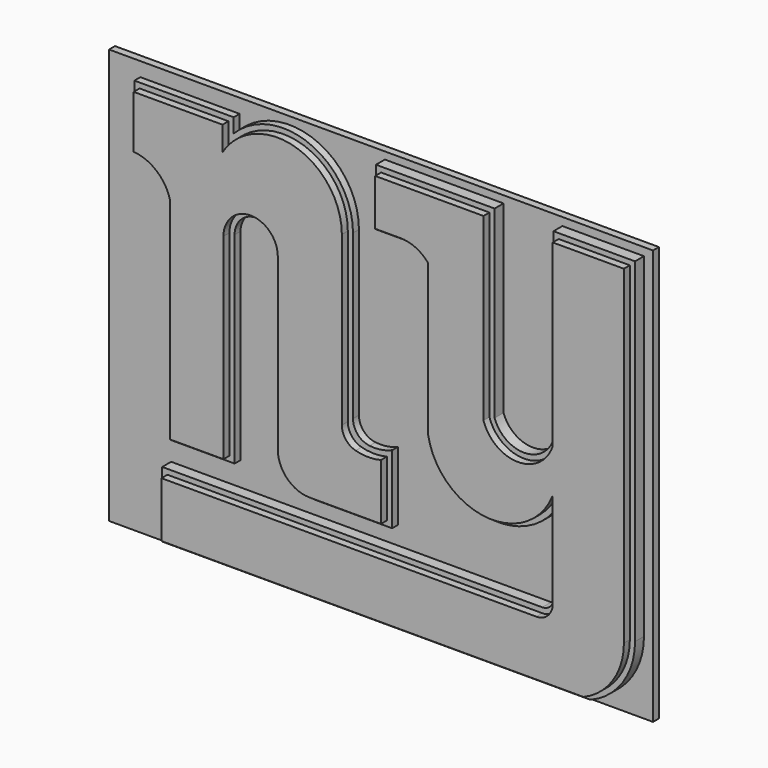
from build123d import *

# Parameters (mm, degrees)
F1_DEPTH = 3.81
F2_W     = 185.822121799
F2_H     = 141.7885944247
F3_DEPTH = 2.54
F5_DEPTH = 2.54
F7_DEPTH = 2.54
F9_DEPTH = 2.54


# Not quite as in the source:
# - a feature names something its author has since deleted; it is built from what else it names


with BuildPart() as f1:
    # F0 (on Front) → F1 (new body)
    with BuildSketch(Plane.XZ):
        with BuildLine():
            Line((61.8872972369, -59.9267967045), (-67.9568648338, -59.9267967045))
            Line((-67.9568648338, -59.9267967045), (-67.9568648338, -82.3878794909))
            Line((-67.9568648338, -82.3878794909), (78.2999321818, -82.3878794909))
            ThreePointArc((78.2999321818, -82.3878794909), (89.3836158058, -73.5038786726), (93.5593023896, -59.9267967045))
            Line((93.5593023896, -59.9267967045), (93.5593023896, 54.4298999012))
            Line((93.5593023896, 54.4298999012), (65.6972972369, 54.4298999012))
            Line((65.6972972369, 54.4298999012), (65.6972972369, -8.2891006023))
            ThreePointArc((65.6972972369, -8.2891006023), (55.6403416055, -15.4575892654), (45.5833859742, -8.2891006023))
            Line((45.5833859742, -8.2891006023), (45.5833859742, 54.7044351697))
            Line((45.5833859742, 54.7044351697), (5.0396709703, 54.7044351697))
            Line((5.0396709703, 54.7044351697), (5.0396709703, 35.2702587843))
            Line((5.0396709703, 35.2702587843), (15.4831645885, 35.2702587843))
            ThreePointArc((15.4831645885, 35.2702587843), (19.6591632782, 34.3958519091), (23.1335591525, 31.9195389748))
            Line((23.1335591525, 31.9195389748), (23.1335591525, -17.3360444605))
            Line((23.1335591525, -17.3360444605), (23.1335591525, -19.20456164))
            ThreePointArc((23.1335591525, -19.20456164), (40.879363735, -38.4902332098), (65.6972972369, -30.0687793642))
            Line((65.6972972369, -30.0687793642), (65.6972972369, -56.1167967045))
            ThreePointArc((65.6972972369, -56.1167967045), (64.5813740732, -58.8108735409), (61.8872972369, -59.9267967045))
        make_face()
        with BuildLine():
            ThreePointArc((23.1335591525, -17.3360444605), (23.1145151518, -18.2703030503), (23.1335591525, -19.20456164))
            Line((23.1335591525, -19.20456164), (23.1335591525, -17.3360444605))
        make_face()
    extrude(amount=F1_DEPTH)

    # F8 (on face) → F9 (join)
    with BuildSketch(Plane.XZ.offset(3.81)):
        with BuildLine():
            Line((67.4725060976, -23.4798739041), (67.4725060976, -56.1167967045))
            ThreePointArc((67.4725060976, -56.1167967045), (65.8366362966, -60.0661357642), (61.8872972369, -61.7020055652))
            Line((61.8872972369, -61.7020055652), (-66.1816559732, -61.7020055652))
            Line((-66.1816559732, -61.7020055652), (-66.1816559732, -80.6126706302))
            Line((-66.1816559732, -80.6126706302), (77.9542927434, -80.6126706302))
            ThreePointArc((77.9542927434, -80.6126706302), (88.0081874746, -72.3683477517), (91.784093529, -59.9267967045))
            Line((91.784093529, -59.9267967045), (91.784093529, 52.6546910405))
            Line((91.784093529, 52.6546910405), (67.4725060976, 52.6546910405))
            Line((67.4725060976, 52.6546910405), (67.4725060976, -8.5750017462))
            ThreePointArc((67.4725060976, -8.5750017462), (55.6403416055, -17.2327981261), (43.8081771135, -8.5750017462))
            Line((43.8081771135, -8.5750017462), (43.8081771135, 52.9292263091))
            Line((43.8081771135, 52.9292263091), (6.8148798309, 52.9292263091))
            Line((6.8148798309, 52.9292263091), (6.8148798309, 37.0454676449))
            Line((6.8148798309, 37.0454676449), (15.4831645885, 37.0454676449))
            ThreePointArc((15.4831645885, 37.0454676449), (20.6976230432, 35.8732781186), (24.9087680131, 32.5822504214))
            Line((24.9087680131, 32.5822504214), (24.9087680131, -17.3729597743))
            ThreePointArc((24.9087680131, -17.3729597743), (24.8898523858, -18.1966120898), (24.9030282278, -19.0203762156))
            ThreePointArc((24.9030282278, -19.0203762156), (44.5022080749, -37.3401368279), (67.4725060976, -23.4798739041))
        make_face()
    extrude(amount=F9_DEPTH)


with BuildPart() as f3:
    # F2 (on face) → F3 (new body)
    with BuildSketch(Plane(origin=(0, 0, 0), x_dir=(-1, 0, 0), z_dir=(0, 1, 0))):
        with Locations((-3.7357322872, -13.7389265001)):
            Rectangle(F2_W, F2_H)
    extrude(amount=F3_DEPTH)

    # F4 (on face) → F5 (join)
    with BuildSketch(Plane.XZ):
        with BuildLine():
            Line((-66.1017629318, 21.9844542444), (-66.1017629318, -51.7266206443))
            Line((-66.1017629318, -51.7266206443), (-44.2493627779, -51.7266206443))
            Line((-44.2493627779, -51.7266206443), (-44.2493627779, 17.092127353))
            ThreePointArc((-44.2493627779, 17.092127353), (-36.7477941327, 24.5936959982), (-29.2462254874, 17.092127353))
            Line((-29.2462254874, 17.092127353), (-29.2462254874, -40.983552891))
            ThreePointArc((-29.2462254874, -40.983552891), (-25.5264816085, -49.9638090121), (-16.5462254874, -53.683552891))
            Line((-16.5462254874, -53.683552891), (9.566242341, -53.683552891))
            Line((9.566242341, -53.683552891), (9.566242341, -30.2003771067))
            ThreePointArc((9.566242341, -30.2003771067), (5.7901732638, -31.2942255388), (1.8598167011, -31.380824371))
            ThreePointArc((1.8598167011, -31.380824371), (-2.1819158801, -29.3091628597), (-3.8061193191, -25.0677778425))
            Line((-3.8061193191, -25.0677778425), (-3.8061193191, 30.7906456292))
            ThreePointArc((-3.8061193191, 30.7906456292), (-18.6015771181, 52.8067259199), (-44.5755193941, 47.4245622754))
            Line((-44.5755193941, 47.4245622754), (-44.5755193941, 52.3168891668))
            Line((-44.5755193941, 52.3168891668), (-78.4956621937, 52.3168891668))
            Line((-78.4956621937, 52.3168891668), (-78.4956621937, 30.7906456292))
            ThreePointArc((-78.4956621937, 30.7906456292), (-70.7684925993, 28.5411928963), (-66.1017629318, 21.9844542444))
        make_face()
    extrude(amount=F5_DEPTH)

    # F6 (on face) → F7 (join)
    with BuildSketch(Plane.XZ.offset(2.54)):
        with BuildLine():
            Line((-76.7176621937, 50.5388891668), (-76.7176621937, 32.5374547699))
            ThreePointArc((-76.7176621937, 32.5374547699), (-68.8934526322, 29.3403456584), (-64.3237629318, 22.2299520002))
            Line((-64.3237629318, 22.2299520002), (-64.3237629318, -49.9486206443))
            Line((-64.3237629318, -49.9486206443), (-46.0273627779, -49.9486206443))
            Line((-46.0273627779, -49.9486206443), (-46.0273627779, 17.092127353))
            ThreePointArc((-46.0273627779, 17.092127353), (-36.7477941327, 26.3716959982), (-27.4682254874, 17.092127353))
            Line((-27.4682254874, 17.092127353), (-27.4682254874, -40.983552891))
            ThreePointArc((-27.4682254874, -40.983552891), (-24.2692457516, -48.7065731551), (-16.5462254874, -51.905552891))
            Line((-16.5462254874, -51.905552891), (7.788242341, -51.905552891))
            Line((7.788242341, -51.905552891), (7.788242341, -32.6938578527))
            ThreePointArc((7.788242341, -32.6938578527), (3.4584477385, -33.2470515492), (-0.8690068072, -32.6758408003))
            ThreePointArc((-0.8690068072, -32.6758408003), (-4.2691980449, -30.4090810578), (-5.5841193191, -26.5399103165))
            Line((-5.5841193191, -26.5399103165), (-5.5841193191, 30.7906456292))
            ThreePointArc((-5.5841193191, 30.7906456292), (-21.6228421821, 51.9676094036), (-46.3535193941, 42.2671954734))
            Line((-46.3535193941, 42.2671954734), (-46.3535193941, 50.5388891668))
            Line((-46.3535193941, 50.5388891668), (-76.7176621937, 50.5388891668))
        make_face()
    extrude(amount=F7_DEPTH)


solid = Compound([f1.part, f3.part])
